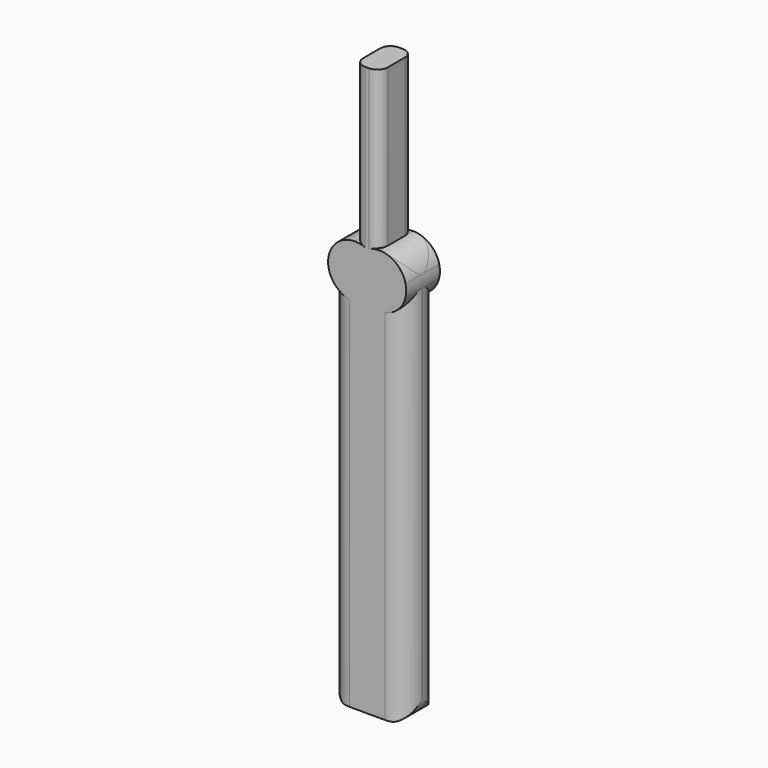
from build123d import *

# Parameters (mm, degrees)
F1_DEPTH     = 10.16
F2_T4_DEPTH  = 50.4313390776
F2_S5_R      = 6.4596874697
F2_T6_DEPTH  = 27
F2_T10_DEPTH = 50.4313390776
F2_S11_R     = 6.4596874697
F2_T12_DEPTH = 27
F2_T16_DEPTH = 50.4313390776
F2_S17_R     = 6.4596874697
F2_T18_DEPTH = 27
F2_T22_DEPTH = 50.4313390776
F2_S23_R     = 6.4596874697
F2_T24_DEPTH = 27
F3_T4_DEPTH  = 112.5049829483
F3_S5_R      = 6.4596874697
F3_T6_DEPTH  = 58
F3_T10_DEPTH = 112.5049829483
F3_S11_R     = 6.4596874697
F3_T12_DEPTH = 58
F3_T16_DEPTH = 112.5049829483
F3_S17_R     = 6.4596874697
F3_T18_DEPTH = 58
F3_T22_DEPTH = 112.5049829483
F3_S23_R     = 6.4596874697
F3_T24_DEPTH = 58


# Not quite as in the source:
# - a fillet or chamfer that OpenCascade refuses, or shapes differently, is made with other operations: its cross-section is extruded or revolved along the edge and cut away or added


with BuildPart() as f1:
    # F0 (on Front) → F1 (new body)
    with BuildSketch(Plane.XZ):
        with BuildLine():
            Line((-2.9818282316, 88.7313390776), (-2.9818282316, 50.8))
            ThreePointArc((-2.9818282316, 50.8), (-8.0369643669, 48.3618993886), (-9.2761479318, 42.8880378604))
            Line((-9.2761479318, 42.8880378604), (-9.2761479318, -44.6169450879))
            ThreePointArc((-9.2761479318, -44.6169450879), (-8.3117384594, -47.249729254), (-5.874895025, -48.6366078258))
            Line((-5.874895025, -48.6366078258), (0, -48.6366078258))
            Line((0, -48.6366078258), (5.874895025, -48.6366078258))
            ThreePointArc((5.874895025, -48.6366078258), (8.3117384594, -47.249729254), (9.2761479318, -44.6169450879))
            Line((9.2761479318, -44.6169450879), (9.2761479318, 42.8880378604))
            ThreePointArc((9.2761479318, 42.8880378604), (8.0369643669, 48.3618993886), (2.9818282316, 50.8))
            Line((2.9818282316, 50.8), (2.9818282316, 88.7313390776))
            Line((2.9818282316, 88.7313390776), (-2.9818282316, 88.7313390776))
        make_face()
    extrude(amount=F1_DEPTH)

    # F2: fillet of radius 2.5 on 4 edges, made by hand


with BuildPart() as f2_tool2:
    # F2_s3 → F2_t4 (new body)
    with BuildSketch(Plane.XY.offset(94.9813390776)):
        with BuildLine():
            ThreePointArc((-0.4818282316, 0), (-2.2495951845, -0.732233047), (-2.9818282316, -2.5))
            Line((-2.9818282316, -2.5), (-2.9818282316, 0))
            Line((-2.9818282316, 0), (-0.4818282316, 0))
        make_face()
    extrude(amount=-F2_T4_DEPTH)

    # F2_s5 → F2_t6 (cut, symmetric)
    with BuildSketch(Plane.XZ.offset(1.2)):
        with Locations((-2.9818282316, 44.3403125303)):
            Circle(F2_S5_R)
    extrude(amount=F2_T6_DEPTH, both=True, mode=Mode.SUBTRACT)


with BuildPart() as f1_1:
    add(f1.part)

    # F2_t1: cut F2_tool2
    add(f2_tool2.part, mode=Mode.SUBTRACT)


with BuildPart() as f2_tool8:
    # F2_s9 → F2_t10 (new body)
    with BuildSketch(Plane.XY.offset(44.55)):
        with BuildLine():
            ThreePointArc((0.4818282316, -10.16), (2.2495951845, -9.427766953), (2.9818282316, -7.66))
            Line((2.9818282316, -7.66), (2.9818282316, -10.16))
            Line((2.9818282316, -10.16), (0.4818282316, -10.16))
        make_face()
    extrude(amount=F2_T10_DEPTH)

    # F2_s11 → F2_t12 (cut, symmetric)
    with BuildSketch(Plane.XZ.offset(8.9)):
        with Locations((2.9818282316, 44.3403125303)):
            Circle(F2_S11_R)
    extrude(amount=F2_T12_DEPTH, both=True, mode=Mode.SUBTRACT)


with BuildPart() as f1_2:
    add(f1_1.part)

    # F2_t7: cut F2_tool8
    add(f2_tool8.part, mode=Mode.SUBTRACT)


with BuildPart() as f2_tool14:
    # F2_s15 → F2_t16 (new body)
    with BuildSketch(Plane.XY.offset(94.9813390776)):
        with BuildLine():
            ThreePointArc((-0.4818282316, -10.16), (-2.2495951845, -9.427766953), (-2.9818282316, -7.66))
            Line((-2.9818282316, -7.66), (-2.9818282316, -10.16))
            Line((-2.9818282316, -10.16), (-0.4818282316, -10.16))
        make_face()
    extrude(amount=-F2_T16_DEPTH)

    # F2_s17 → F2_t18 (cut, symmetric)
    with BuildSketch(Plane.XZ.offset(8.9)):
        with Locations((-2.9818282316, 44.3403125303)):
            Circle(F2_S17_R)
    extrude(amount=F2_T18_DEPTH, both=True, mode=Mode.SUBTRACT)


with BuildPart() as f1_3:
    add(f1_2.part)

    # F2_t13: cut F2_tool14
    add(f2_tool14.part, mode=Mode.SUBTRACT)


with BuildPart() as f2_tool20:
    # F2_s21 → F2_t22 (new body)
    with BuildSketch(Plane.XY.offset(44.55)):
        with BuildLine():
            ThreePointArc((0.4818282316, 0), (2.2495951845, -0.732233047), (2.9818282316, -2.5))
            Line((2.9818282316, -2.5), (2.9818282316, 0))
            Line((2.9818282316, 0), (0.4818282316, 0))
        make_face()
    extrude(amount=F2_T22_DEPTH)

    # F2_s23 → F2_t24 (cut, symmetric)
    with BuildSketch(Plane.XZ.offset(1.2)):
        with Locations((2.9818282316, 44.3403125303)):
            Circle(F2_S23_R)
    extrude(amount=F2_T24_DEPTH, both=True, mode=Mode.SUBTRACT)


with BuildPart() as f1_4:
    add(f1_3.part)

    # F2_t19: cut F2_tool20
    add(f2_tool20.part, mode=Mode.SUBTRACT)

    # F3: fillet of radius 5 on 4 edges, made by hand


with BuildPart() as f3_tool2:
    # F3_s3 → F3_t4 (new body)
    with BuildSketch(Plane.XY.offset(55.3880378604)):
        with BuildLine():
            ThreePointArc((-4.2761479318, 0), (-7.8116818377, -1.4644660941), (-9.2761479318, -5))
            Line((-9.2761479318, -5), (-9.2761479318, 0))
            Line((-9.2761479318, 0), (-4.2761479318, 0))
        make_face()
    extrude(amount=-F3_T4_DEPTH)

    # F3_s5 → F3_t6 (cut, symmetric)
    with BuildSketch(Plane.XZ.offset(2.5)):
        with Locations((-2.9818282316, 44.3403125303)):
            Circle(F3_S5_R)
    extrude(amount=F3_T6_DEPTH, both=True, mode=Mode.SUBTRACT)


with BuildPart() as f1_5:
    add(f1_4.part)

    # F3_t1: cut F3_tool2
    add(f3_tool2.part, mode=Mode.SUBTRACT)


with BuildPart() as f3_tool8:
    # F3_s9 → F3_t10 (new body)
    with BuildSketch(Plane.XY.offset(-57.1169450879)):
        with BuildLine():
            ThreePointArc((4.2761479318, 0), (7.8116818377, -1.4644660941), (9.2761479318, -5))
            Line((9.2761479318, -5), (9.2761479318, 0))
            Line((9.2761479318, 0), (4.2761479318, 0))
        make_face()
    extrude(amount=F3_T10_DEPTH)

    # F3_s11 → F3_t12 (cut, symmetric)
    with BuildSketch(Plane.XZ.offset(2.5)):
        with Locations((2.9818282316, 44.3403125303)):
            Circle(F3_S11_R)
    extrude(amount=F3_T12_DEPTH, both=True, mode=Mode.SUBTRACT)


with BuildPart() as f1_6:
    add(f1_5.part)

    # F3_t7: cut F3_tool8
    add(f3_tool8.part, mode=Mode.SUBTRACT)


with BuildPart() as f3_tool14:
    # F3_s15 → F3_t16 (new body)
    with BuildSketch(Plane.XY.offset(55.3880378604)):
        with BuildLine():
            ThreePointArc((-4.2761479318, -10.16), (-7.8116818377, -8.6955339059), (-9.2761479318, -5.16))
            Line((-9.2761479318, -5.16), (-9.2761479318, -10.16))
            Line((-9.2761479318, -10.16), (-4.2761479318, -10.16))
        make_face()
    extrude(amount=-F3_T16_DEPTH)

    # F3_s17 → F3_t18 (cut, symmetric)
    with BuildSketch(Plane.XZ.offset(7.7)):
        with Locations((-2.9818282316, 44.3403125303)):
            Circle(F3_S17_R)
    extrude(amount=F3_T18_DEPTH, both=True, mode=Mode.SUBTRACT)


with BuildPart() as f1_7:
    add(f1_6.part)

    # F3_t13: cut F3_tool14
    add(f3_tool14.part, mode=Mode.SUBTRACT)


with BuildPart() as f3_tool20:
    # F3_s21 → F3_t22 (new body)
    with BuildSketch(Plane.XY.offset(-57.1169450879)):
        with BuildLine():
            ThreePointArc((4.2761479318, -10.16), (7.8116818377, -8.6955339059), (9.2761479318, -5.16))
            Line((9.2761479318, -5.16), (9.2761479318, -10.16))
            Line((9.2761479318, -10.16), (4.2761479318, -10.16))
        make_face()
    extrude(amount=F3_T22_DEPTH)

    # F3_s23 → F3_t24 (cut, symmetric)
    with BuildSketch(Plane.XZ.offset(7.7)):
        with Locations((2.9818282316, 44.3403125303)):
            Circle(F3_S23_R)
    extrude(amount=F3_T24_DEPTH, both=True, mode=Mode.SUBTRACT)


with BuildPart() as f1_8:
    add(f1_7.part)

    # F3_t19: cut F3_tool20
    add(f3_tool20.part, mode=Mode.SUBTRACT)


solid = f1_8.part
